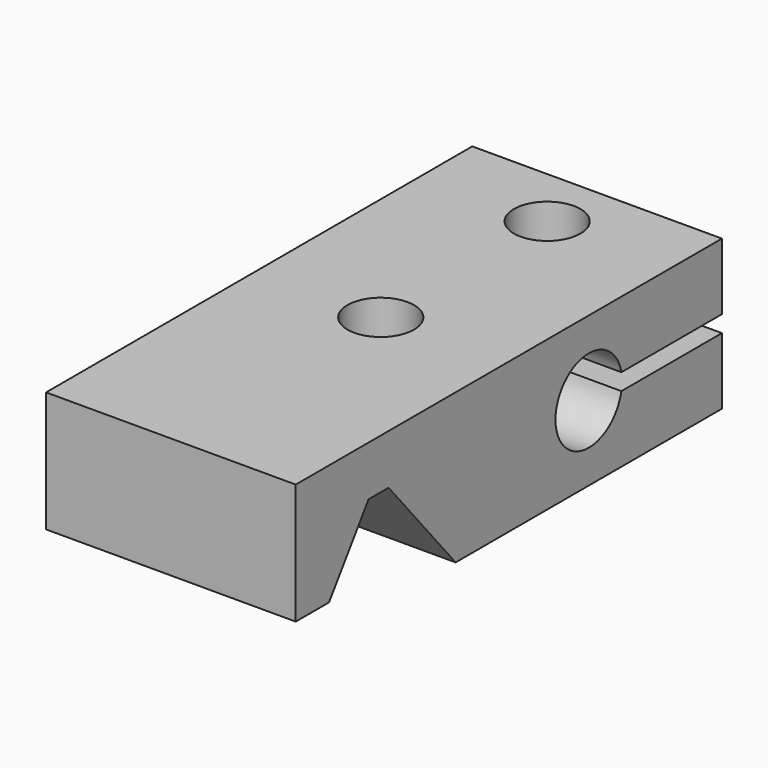
from build123d import *

# Parameters (mm, degrees)
F1_DEPTH = 30
F3_W     = 19.6464200949
F3_H     = 2
F4_DEPTH = 30.001
F2_R     = 5
F5_DEPTH = 30.001
F6_R     = 4
F7_DEPTH = 18.001
F8_DEPTH = 30.001


# Not quite as in the source:
# - a feature names something its author has since deleted; it is built from what else it names


with BuildPart() as f1:
    # F0 (on Right) → F1 (new body)
    with BuildSketch(Plane.YZ):
        Polygon((13.9517640748, 20.9442070276), (24.0209596489, 8.9442070276), (64.0209596489, 8.9442070276), (64.0209596489, 26.9442070276), (0, 26.9442070276), (0, 12.4442070276), (5, 12.4442070276), (10.9517640748, 20.9442070276), align=None)
    extrude(amount=F1_DEPTH)

    # F3 (on face) → F4 (cut, through all)
    with BuildSketch(Plane.YZ.offset(30)):
        with Locations((56.7216197717, 17.9442070276)):
            Rectangle(F3_W, F3_H)
    extrude(amount=-F4_DEPTH, mode=Mode.SUBTRACT)

    # F2 (on face) → F5 (cut, through all)
    with BuildSketch(Plane.YZ.offset(30)):
        with Locations((44.0209596489, 17.9442070276)):
            Circle(F2_R)
    extrude(amount=-F5_DEPTH, mode=Mode.SUBTRACT)

    # F6 (on face) → F7 (cut, through all)
    with BuildSketch(Plane.XY.offset(26.9442070276)):
        with Locations((15, 31.5209596489)):
            Circle(F6_R)
        with Locations((15, 56.5209596489)):
            Circle(F6_R)
    extrude(amount=-F7_DEPTH, mode=Mode.SUBTRACT)

    # F2 (on face) → F8 (cut, through all)
    with BuildSketch(Plane.YZ.offset(30)):
        with Locations((44.0209596489, 17.9442070276)):
            Circle(F2_R)
    extrude(amount=-F8_DEPTH, mode=Mode.SUBTRACT)


solid = f1.part
